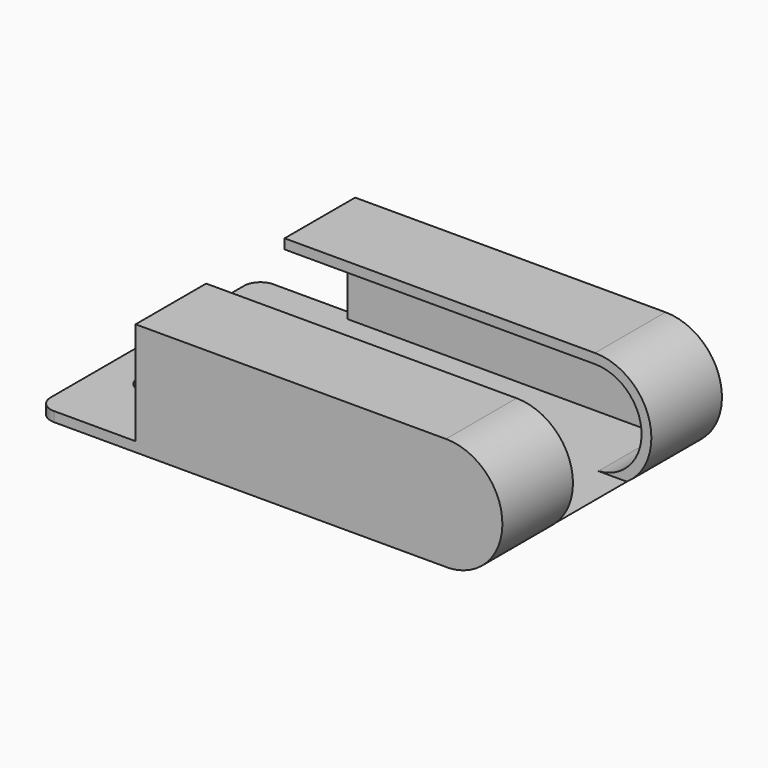
from build123d import *

# Parameters (mm, degrees)
F1_DEPTH       = 42
F1_DEPTH_BACK  = 42
F3_DEPTH       = 3
F4_W           = 171.0703811337
F4_H           = 30
F5_DEPTH       = 31.501
F6_R           = 5
F8_D           = 5
F8_CSINK_D     = 10
F8_CSINK_ANGLE = 90


# Not quite as in the source:
# - a pattern or mirror of a feature is missing from the dataset's text; its kind, count and spacing are read off the source's solid


with BuildPart() as f1:
    # F0 (on Front) → F1 (new body, two sides)
    with BuildSketch(Plane.XZ) as f1_sk:
        with BuildLine():
            Line((-74.8302465006, 17.25), (-74.8302465006, 14.25))
            Line((-74.8302465006, 14.25), (20.1697534994, 14.25))
            ThreePointArc((20.1697534994, 14.25), (34.429081055, 0.4973529093), (21.2011066634, -14.25))
            Line((21.2011066634, -14.25), (-104.8302465006, -14.25))
            Line((-104.8302465006, -14.25), (-104.8302465006, -17.25))
            Line((-104.8302465006, -17.25), (21.3044886882, -17.25))
            ThreePointArc((21.3044886882, -17.25), (37.4290815856, 0.5490131867), (20.1697534994, 17.25))
            Line((20.1697534994, 17.25), (-74.8302465006, 17.25))
        make_face()
    extrude(amount=F1_DEPTH)
    extrude(f1_sk.sketch, amount=-F1_DEPTH_BACK)

    # F2 (on face) → F3 (join)
    with BuildSketch(Plane.XZ.offset(42)):
        with BuildLine():
            Line((20.1697534994, 17.25), (-74.8302465006, 17.25))
            Line((-74.8302465006, 17.25), (-74.8302465006, -17.25))
            Line((-74.8302465006, -17.25), (21.3044886882, -17.25))
            ThreePointArc((21.3044886882, -17.25), (37.4290815856, 0.5490131867), (20.1697534994, 17.25))
        make_face()
    f3 = extrude(amount=-F3_DEPTH)

    # F3_copies: F3 across plane
    add(f3.mirror(Plane.ZX))

    # F4 (on face) → F5 (cut, through all)
    with BuildSketch(Plane.XY.offset(-14.25)):
        with Locations((-19.9944982305, 0)):
            Rectangle(F4_W, F4_H)
    extrude(amount=F5_DEPTH, mode=Mode.SUBTRACT)

    # F6
    f6_edges = [f1.edges().sort_by_distance(p)[0] for p in [
        (-104.830247, -42, -15.75),
        (-104.830247, 42, -15.75),
    ]]
    fillet(f6_edges, radius=F6_R)

    # F8 (through all)
    with Locations(Plane.XY.offset(-14.25)):
        with Locations((-89.8302465006, -16.0900652409), (-89.8302465006, 16.0900652409), (0, 0)):
            CounterSinkHole(F8_D / 2, F8_CSINK_D / 2, counter_sink_angle=F8_CSINK_ANGLE)


solid = f1.part
